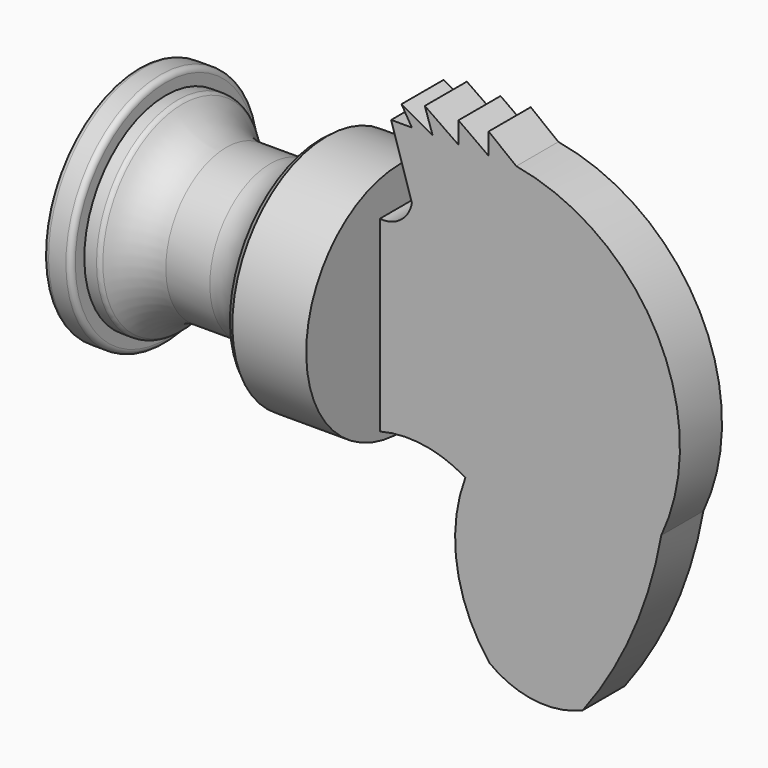
from build123d import *

# Parameters (mm, degrees)
F4_R     = 0.508
F7_DEPTH = 2.54


# Not quite as in the source:
# - a fillet or chamfer that OpenCascade refuses, or shapes differently, is made with other operations: its cross-section is extruded or revolved along the edge and cut away or added


with BuildPart() as f1:
    # F0 (on Front) → F1 (revolve)
    with BuildSketch(Plane.XZ):
        Polygon((-25.4, 0), (0, 0), (0, 11.43), (-7.62, 11.43), (-7.62, 7.3114731075), (-20.32, 7.3114731075), (-21.2499899719, 9.835730216), (-22.7114037935, 9.835730216), (-22.7114037935, 11.43), (-25.4, 11.43), align=None)
    revolve(axis=Axis((-12.7, 0, 0), (-1, 0, 0)))

    # F2: fillet of radius 5.08 on 1 edges, made by hand

    # F2_s1 → F2_t2 (revolve)
    with BuildSketch(Plane.XZ):
        with BuildLine():
            ThreePointArc((-16.8597077176, 7.3114731075), (-19.3918240371, 7.9875218198), (-21.2499899719, 9.835730216))
            Line((-21.2499899719, 9.835730216), (-20.32, 7.3114731075))
            Line((-20.32, 7.3114731075), (-16.8597077176, 7.3114731075))
        make_face()
    revolve(axis=Axis((-20.32, 0, 0), (-1, 0, 0)))

    # F3: fillet of radius 5.08 on 1 edges, made by hand

    # F3_s1 → F3_t2 (revolve)
    with BuildSketch(Plane.XZ):
        with BuildLine():
            ThreePointArc((-7.62, 11.43), (-9.3738270483, 8.4741600369), (-12.6081829822, 7.3114731075))
            Line((-12.6081829822, 7.3114731075), (-7.62, 7.3114731075))
            Line((-7.62, 7.3114731075), (-7.62, 11.43))
        make_face()
    revolve(axis=Axis((-7.62, 0, 0), (-1, 0, 0)))

    # F4
    f4_edges = [f1.edges().sort_by_distance(p)[0] for p in [
        (-21.24999, 0, -9.83573),
        (-22.711404, 0, -11.43),
        (-25.4, 0, -11.43),
    ]]
    fillet(f4_edges, radius=F4_R)

    # F5: chamfer of 0.508 on 1 edges, made by hand

    # F5_s1 → F5_t2 (revolve, cut)
    with BuildSketch(Plane.XZ):
        with BuildLine():
            Line((-7.7429817287, 10.9728511125), (-7.1192910196, 11.442218632))
            Line((-7.1192910196, 11.442218632), (-7.1192910196, 11.452378632))
            ThreePointArc((-7.1192910196, 11.452378632), (-7.3696455098, 11.44016), (-7.62, 11.44016))
            Line((-7.62, 11.44016), (-7.629976366, 11.4319229462))
            ThreePointArc((-7.629976366, 11.4319229462), (-7.6800748035, 11.2010835053), (-7.7527446032, 10.9756639192))
            Line((-7.7527446032, 10.9756639192), (-7.7429817287, 10.9728511125))
        make_face()
    revolve(axis=Axis((-7.62, 0, 0), (-1, 0, 0)), mode=Mode.SUBTRACT)

    # F6 (on Front) → F7 (join, symmetric)
    with BuildSketch(Plane.XZ):
        with BuildLine():
            ThreePointArc((3.0916559044, 10.094515048), (2.0073718485, 8.3160562532), (0, 7.7601373196))
            Line((0, 7.7601373196), (0, -10.331296362))
            ThreePointArc((0, -10.331296362), (4.2573596526, -10.1174017701), (8.2606375217, -11.5818567574))
            ThreePointArc((8.2606375217, -11.5818567574), (7.4512752544, -19.3926799341), (10.5950161815, -26.5885759145))
            ThreePointArc((10.5950161815, -26.5885759145), (14.9502413437, -28.3499722326), (19.5990465581, -27.6723932475))
            ThreePointArc((19.5990465581, -27.6723932475), (24.422816729, -19.452646971), (27.1857772022, -10.331296362))
            ThreePointArc((27.1857772022, -10.331296362), (26.8307486913, 6.5599572314), (13.1795061752, 16.5140554309))
            Line((13.1795061752, 16.5140554309), (10.5116451159, 18.5983236879))
            Line((10.5116451159, 18.5983236879), (10.5116451159, 16.5140554309))
            Line((10.5116451159, 16.5140554309), (7.5936717913, 18.5983236879))
            Line((7.5936717913, 18.5983236879), (7.5936717913, 16.5140554309))
            Line((7.5936717913, 16.5140554309), (4.342216067, 18.7650639564))
            Line((4.342216067, 18.7650639564), (5.0925519317, 16.5140554309))
            Line((5.0925519317, 16.5140554309), (2.0912080654, 18.1814711541))
            Line((2.0912080654, 18.1814711541), (3.0916559044, 16.5140554309))
            Line((3.0916559044, 16.5140554309), (1.0907602264, 16.5140554309))
            Line((1.0907602264, 16.5140554309), (3.0916559044, 10.094515048))
        make_face()
    extrude(amount=F7_DEPTH, both=True)


solid = f1.part
